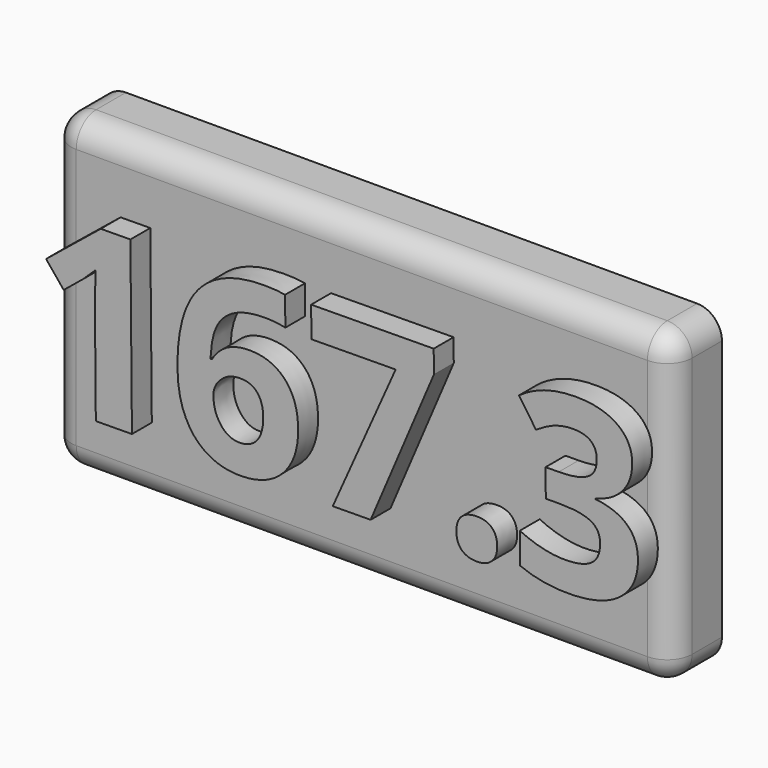
from build123d import *

# Parameters (mm, degrees)
F0_W         = 50
F0_H         = 25
F1_DEPTH     = 5
F3_R         = 2
F2_TEXT_SIZE = 19.2713038241
F4_DEPTH     = 2


# Not quite as in the source:
# - Text() gives the source's letters only with a copy of the font that has no kerning and outlines rounded to 1/6400 em; it was checked with that copy


with BuildPart() as f1:
    # F0 (on Front) → F1 (new body)
    with BuildSketch(Plane.XZ):
        Rectangle(F0_W, F0_H)
    extrude(amount=F1_DEPTH)

    # F3
    f3_edges = [f1.edges().sort_by_distance(p)[0] for p in [
        (25, -5, 0),
        (0, -5, 12.5),
        (-25, -5, 0),
        (0, -5, -12.5),
        (-25, -2.5, 12.5),
        (25, -2.5, 12.5),
        (25, -2.5, -12.5),
        (-25, -2.5, -12.5),
    ]]
    fillet(f3_edges, radius=F3_R)

    # F2 (on face) → F4 (join)
    with BuildSketch(Plane.XZ.offset(5)):
        with Locations(Location((-24.874369891, -6.9610827154), (0, 0, 0.5146105552))):
            Text('167.3', F2_TEXT_SIZE, font='Open Sans', font_style=FontStyle.BOLD, text_align=(TextAlign.LEFT, TextAlign.BOTTOM))
    extrude(amount=F4_DEPTH)


solid = f1.part
